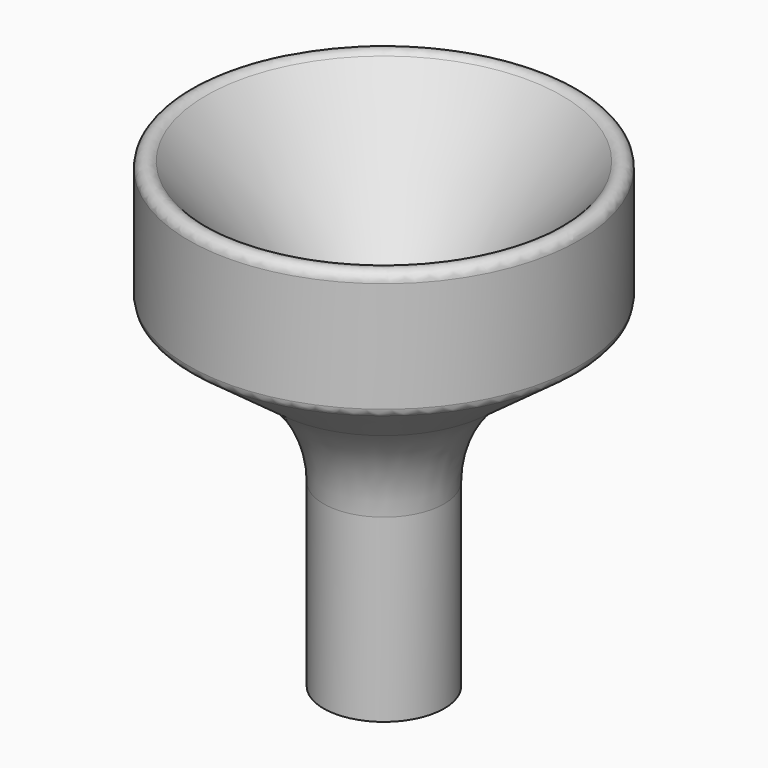
from build123d import *

# Parameters (mm, degrees)
F2_R = 2.54


with BuildPart() as f1:
    # F0 (on Front) → F1 (revolve)
    with BuildSketch(Plane.XZ):
        with BuildLine():
            Line((50.4768975079, 61.4194460213), (0, 0))
            Line((0, 0), (0, -63.5373517871))
            Line((0, -63.5373517871), (15.5935517171, -63.5373517871))
            Line((15.5935517171, -63.5373517871), (15.5935517171, -16.9645253417))
            ThreePointArc((15.5935517171, -16.9645253417), (18.9662168832, -2.8402970726), (28.3564869314, 8.2363234833))
            Line((28.3564869314, 8.2363234833), (50.4768975079, 24.4736485183))
            Line((50.4768975079, 24.4736485183), (50.4768975079, 61.4194460213))
        make_face()
    revolve(axis=Axis((0, 0, 22.0490116626), (0, 0, 1)))

    # F2
    f2_edges = [f1.edges().sort_by_distance(p)[0] for p in [
        (-50.476898, 0, 61.419446),
        (-50.476898, 0, 24.473649),
    ]]
    fillet(f2_edges, radius=F2_R)


solid = f1.part
